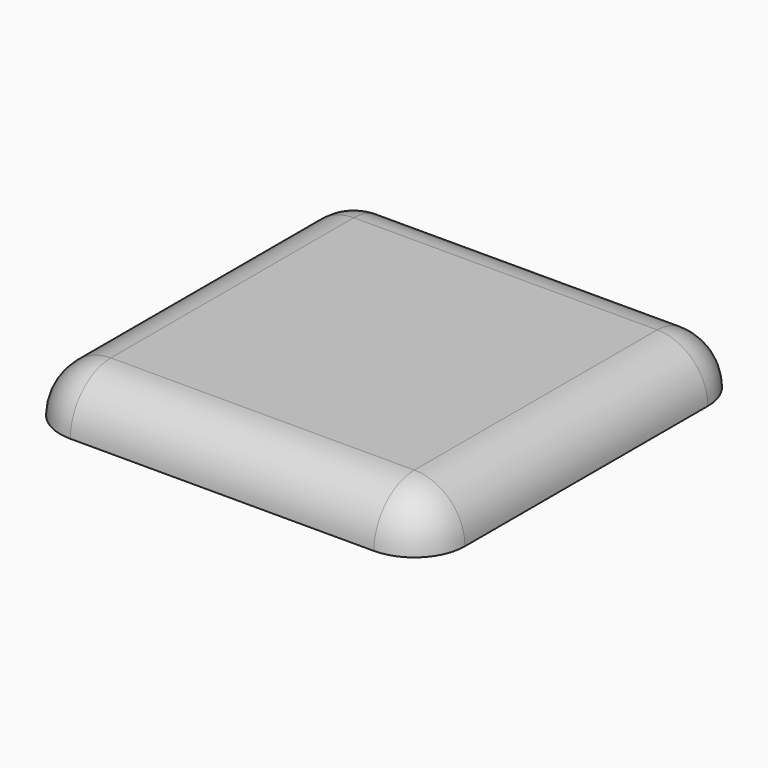
from build123d import *

# Parameters (mm, degrees)
F0_W     = 20
F0_H     = 20
F1_DEPTH = 2.5
F2_R     = 2.49999


# Not quite as in the source:
# - a fillet or chamfer is up to 0.001 mm smaller than in the source, because OpenCascade refuses the exact size


with BuildPart() as f1:
    # F0 (on Top) → F1 (new body)
    with BuildSketch(Plane.XY):
        Rectangle(F0_W, F0_H)
    extrude(amount=F1_DEPTH)

    # F2 (radius 2.5 in the source; OpenCascade refuses exactly that, so slightly less here)
    f2_edges = [f1.edges().sort_by_distance(p)[0] for p in [
        (10, -10, 1.25),
        (10, 10, 1.25),
        (-10, -10, 1.25),
        (-10, 10, 1.25),
        (0, -10, 2.5),
        (10, 0, 2.5),
        (0, 10, 2.5),
        (-10, 0, 2.5),
    ]]
    fillet(f2_edges, radius=F2_R)


solid = f1.part
